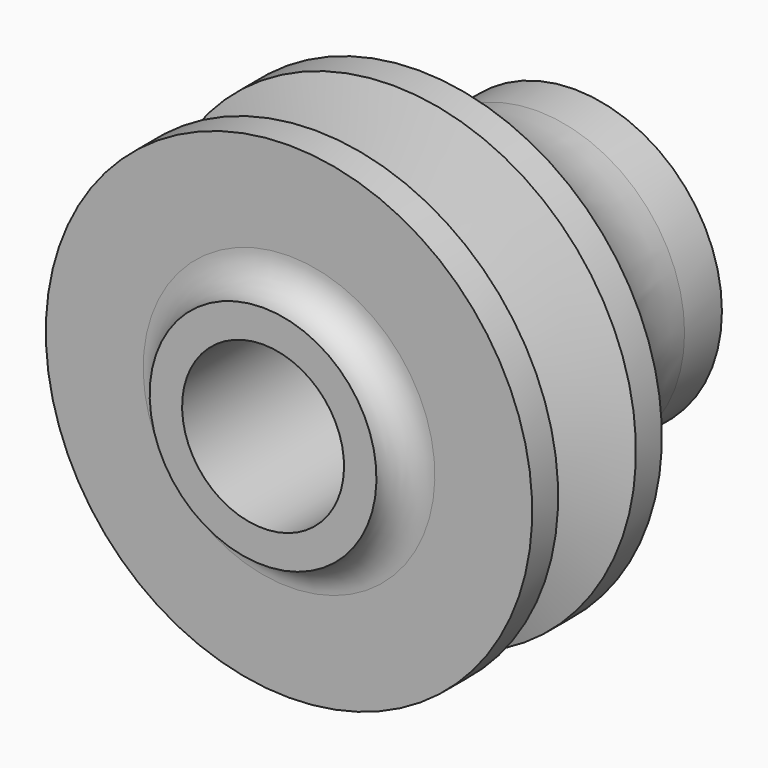
from build123d import *

# Parameters (mm, degrees)
F3_R = 0.99999


# Not quite as in the source:
# - a fillet or chamfer that OpenCascade refuses, or shapes differently, is made with other operations: its cross-section is extruded or revolved along the edge and cut away or added
# - a fillet or chamfer is up to 0.001 mm smaller than in the source, because OpenCascade refuses the exact size


with BuildPart() as f1:
    # F0 (on Right) → F1 (revolve)
    with BuildSketch(Plane.YZ):
        Polygon((-47.0208749175, 2.497), (-35.0208749175, 2.497), (-35.0208749175, 4.55), (-41.0208749175, 4.55), (-41.0208749175, 7.5), (-42.0208749175, 7.5), (-43.0208749175, 4.55), (-43.5208749175, 4.55), (-44.0208749175, 4.55), (-45.0208749175, 7.5), (-46.0208749175, 7.5), (-46.0208749175, 4.55), (-46.0208749175, 3.497), (-47.0208749175, 3.497), align=None)
    revolve(axis=Axis((0, -14.7727020085, 0), (0, 1, 0)))

    # F2: fillet of radius 5 on 1 edges, made by hand

    # F2_s1 → F2_t2 (revolve)
    with BuildSketch(Plane.YZ):
        with BuildLine():
            ThreePointArc((-36.460447306, 4.55), (-39.1761424288, 5.3517860941), (-41.0208749175, 7.5))
            Line((-41.0208749175, 7.5), (-41.1120834697, 7.459))
            ThreePointArc((-41.1120834697, 7.459), (-41.1208749175, 6.025), (-41.1208749175, 4.55))
            Line((-41.1208749175, 4.55), (-41.0208749175, 4.45))
            Line((-41.0208749175, 4.45), (-36.460447306, 4.45))
            Line((-36.460447306, 4.45), (-36.460447306, 4.55))
        make_face()
    revolve(axis=Axis((0, -41.0208749175, 0), (0, 1, 0)))

    # F3 (radius 1 in the source; OpenCascade refuses exactly that, so slightly less here)
    f3_edges = [f1.edges().sort_by_distance(p)[0] for p in [
        (0, -46.020875, -3.497),
    ]]
    fillet(f3_edges, radius=F3_R)


solid = f1.part
